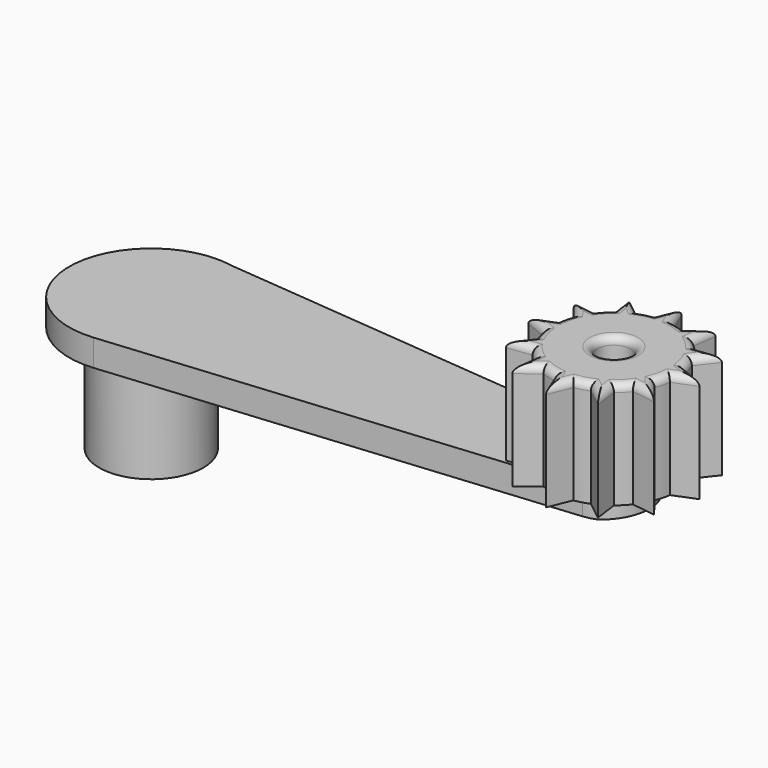
from build123d import *

# Parameters (mm, degrees)
F1_DEPTH = 6.35
F2_R     = 4
F3_DEPTH = 25.4
F5_R     = 12.3831854663
F6_DEPTH = 25.4
F7_R     = 4
F8_DEPTH = 25.4
F9_R     = 1.778


# Not quite as in the source:
# - a fillet or chamfer that OpenCascade refuses, or shapes differently, is made with other operations: its cross-section is extruded or revolved along the edge and cut away or added


with BuildPart() as f1:
    # F0 (on Top) → F1 (new body)
    with BuildSketch(Plane.XY):
        with BuildLine():
            Line((0, 19.5379621843), (3.5827930435, 19.2066540637))
            ThreePointArc((3.5827930435, 19.2066540637), (1.7990394008, 19.4549588422), (0, 19.5379621843))
        make_face()
        with BuildLine():
            Line((110.0876327298, 9.3579360824), (3.5827930435, 19.2066540637))
            Line((3.5827930435, 19.2066540637), (0, 19.5379621843))
            ThreePointArc((0, 19.5379621843), (-19.5168552551, -0.9079247047), (1.813887741, -19.453580071))
            Line((1.8138877409, -19.453580071), (110.0876327298, -9.3579360824))
            ThreePointArc((110.0876327298, -9.3579360824), (118.6201465698, 0), (110.0876327298, 9.3579360824))
        make_face()
    extrude(amount=F1_DEPTH)

    # F2 (on face) → F3 (cut)
    with BuildSketch(Plane.XY.offset(6.35)):
        with Locations((110.0876327298, 0)):
            Circle(F2_R)
    extrude(amount=-F3_DEPTH, mode=Mode.SUBTRACT)

    # F4: chamfer of 5.08 on 1 edges, made by hand

    # F4_s1 → F4_t2 (revolve, cut)
    with BuildSketch(Plane.XZ):
        Polygon((119.1676327298, 0), (114.0876327298, 5.08), (114.0876327298, 0), align=None)
    revolve(axis=Axis((110.0876327298, 0, 0), (0, 0, 1)), mode=Mode.SUBTRACT)

    # F5 (on face) → F6 (join)
    with BuildSketch(Plane(origin=(0, 0, 0), x_dir=(1, 0, 0), z_dir=(0, 0, -1))):
        Circle(F5_R)
    extrude(amount=F6_DEPTH)


with BuildPart() as f8:
    # F7 (on face) → F8 (new body)
    with BuildSketch(Plane.XY.offset(6.35)):
        with BuildLine():
            ThreePointArc((125.0559656513, -2.0569956955), (125.1614333891, -1.0309002972), (125.1966440058, 0))
            ThreePointArc((125.1966440058, 0), (125.1529244508, 1.1485674127), (125.0220188001, 2.2904878178))
            ThreePointArc((125.0220188001, 2.2904878178), (124.6508382593, 4.0243342858), (124.0790871399, 5.7027559329))
            ThreePointArc((124.0790871399, 5.7027559329), (123.1130347073, 7.656443369), (121.8759465477, 9.4508136724))
            ThreePointArc((121.8759465477, 9.4508136724), (120.687571536, 10.7667784895), (119.3532097183, 11.9344587145))
            ThreePointArc((119.3532097183, 11.9344587145), (117.5397400523, 13.143375449), (115.5712051277, 14.0788016356))
            ThreePointArc((115.5712051277, 14.0788016356), (113.8840597698, 14.624273092), (112.1446284253, 14.9683329214))
            ThreePointArc((112.1446284253, 14.9683329214), (109.9696592584, 15.1085506915), (107.797144912, 14.9343860702))
            ThreePointArc((107.797144912, 14.9343860702), (106.0632984441, 14.5632055295), (104.3848767969, 13.99145441))
            ThreePointArc((104.3848767969, 13.99145441), (102.4311893608, 13.0254019775), (100.6368190574, 11.7883138179))
            ThreePointArc((100.6368190574, 11.7883138179), (99.3208542403, 10.5999388062), (98.1531740153, 9.2655769885))
            ThreePointArc((98.1531740153, 9.2655769885), (96.9442572809, 7.4521073225), (96.0088310942, 5.4835723979))
            ThreePointArc((96.0088310942, 5.4835723979), (95.4633596378, 3.79642704), (95.1192998084, 2.0569956955))
            ThreePointArc((95.1192998084, 2.0569956955), (94.9790820383, -0.1179734715), (95.1532466596, -2.2904878178))
            ThreePointArc((95.1532466596, -2.2904878178), (95.5244272003, -4.0243342858), (96.0961783198, -5.7027559329))
            ThreePointArc((96.0961783198, -5.7027559329), (97.0622307523, -7.656443369), (98.299318912, -9.4508136724))
            ThreePointArc((98.299318912, -9.4508136724), (99.4876939236, -10.7667784895), (100.8220557413, -11.9344587145))
            ThreePointArc((100.8220557413, -11.9344587145), (102.6355254073, -13.143375449), (104.604060332, -14.0788016356))
            ThreePointArc((104.604060332, -14.0788016356), (106.2912056898, -14.624273092), (108.0306370343, -14.9683329214))
            ThreePointArc((108.0306370343, -14.9683329214), (110.2056062013, -15.1085506915), (112.3781205476, -14.9343860702))
            ThreePointArc((112.3781205476, -14.9343860702), (114.1119670156, -14.5632055295), (115.7903886627, -13.99145441))
            ThreePointArc((115.7903886627, -13.99145441), (117.7440760988, -13.0254019775), (119.5384464022, -11.7883138179))
            ThreePointArc((119.5384464022, -11.7883138179), (120.8544112194, -10.5999388062), (122.0220914443, -9.2655769885))
            ThreePointArc((122.0220914443, -9.2655769885), (123.2310081788, -7.4521073225), (124.1664343655, -5.4835723979))
            ThreePointArc((124.1664343655, -5.4835723979), (124.7119058218, -3.79642704), (125.0559656513, -2.0569956955))
        make_face()
        with Locations((110.0876327298, 0)):
            Circle(F7_R, mode=Mode.SUBTRACT)
        with BuildLine():
            ThreePointArc((125.0220188001, 2.2904878178), (125.1529244508, 1.1485674127), (125.1966440058, 0))
            ThreePointArc((125.1966440058, 0), (125.1614333891, -1.0309002972), (125.0559656513, -2.0569956955))
            Line((125.0559656513, -2.0569956955), (130.3779385678, 0.0894885204))
            Line((130.3779385678, 0.0894885204), (125.0220188001, 2.2904878178))
        make_face()
        with BuildLine():
            ThreePointArc((121.8759465477, 9.4508136724), (123.1130347073, 7.656443369), (124.0790871399, 5.7027559329))
            Line((124.0790871399, 5.7027559329), (127.6148087759, 10.222652251))
            Line((127.6148087759, 10.222652251), (121.8759465477, 9.4508136724))
        make_face()
        with BuildLine():
            Line((127.7042972963, -10.067653587), (124.1664343655, -5.4835723979))
            ThreePointArc((124.1664343655, -5.4835723979), (123.2310081788, -7.4521073225), (122.0220914443, -9.2655769885))
            Line((122.0220914443, -9.2655769885), (127.7042972963, -10.067653587))
        make_face()
        with BuildLine():
            ThreePointArc((115.5712051277, 14.0788016356), (117.5397400523, 13.143375449), (119.3532097183, 11.9344587145))
            Line((119.3532097183, 11.9344587145), (120.1552863168, 17.6166645665))
            Line((120.1552863168, 17.6166645665), (115.5712051277, 14.0788016356))
        make_face()
        with BuildLine():
            Line((120.3102849809, -17.527176046), (119.5384464022, -11.7883138179))
            ThreePointArc((119.5384464022, -11.7883138179), (117.7440760988, -13.0254019775), (115.7903886627, -13.99145441))
            Line((115.7903886627, -13.99145441), (120.3102849809, -17.527176046))
        make_face()
        with BuildLine():
            ThreePointArc((107.797144912, 14.9343860702), (109.9696592584, 15.1085506915), (112.1446284253, 14.9683329214))
            Line((112.1446284253, 14.9683329214), (109.9981442094, 20.290305838))
            Line((109.9981442094, 20.290305838), (107.797144912, 14.9343860702))
        make_face()
        with BuildLine():
            Line((110.1771212503, -20.290305838), (112.3781205476, -14.9343860702))
            ThreePointArc((112.3781205476, -14.9343860702), (110.2056062013, -15.1085506915), (108.0306370343, -14.9683329214))
            Line((108.0306370343, -14.9683329214), (110.1771212503, -20.290305838))
        make_face()
        with BuildLine():
            ThreePointArc((100.6368190574, 11.7883138179), (102.4311893608, 13.0254019775), (104.3848767969, 13.99145441))
            Line((104.3848767969, 13.99145441), (99.8649804788, 17.527176046))
            Line((99.8649804788, 17.527176046), (100.6368190574, 11.7883138179))
        make_face()
        with BuildLine():
            Line((100.0199791429, -17.6166645665), (104.604060332, -14.0788016356))
            ThreePointArc((104.604060332, -14.0788016356), (102.6355254073, -13.143375449), (100.8220557413, -11.9344587145))
            Line((100.8220557413, -11.9344587145), (100.0199791429, -17.6166645665))
        make_face()
        with BuildLine():
            ThreePointArc((96.0088310942, 5.4835723979), (96.9442572809, 7.4521073225), (98.1531740153, 9.2655769885))
            Line((98.1531740153, 9.2655769885), (92.4709681633, 10.067653587))
            Line((92.4709681633, 10.067653587), (96.0088310942, 5.4835723979))
        make_face()
        with BuildLine():
            Line((92.5604566838, -10.222652251), (98.299318912, -9.4508136724))
            ThreePointArc((98.299318912, -9.4508136724), (97.0622307523, -7.656443369), (96.0961783198, -5.7027559329))
            Line((96.0961783198, -5.7027559329), (92.5604566838, -10.222652251))
        make_face()
        with BuildLine():
            ThreePointArc((95.1532466596, -2.2904878178), (94.9790820383, -0.1179734715), (95.1192998084, 2.0569956955))
            Line((95.1192998084, 2.0569956955), (89.7973268918, -0.0894885204))
            Line((89.7973268918, -0.0894885204), (95.1532466596, -2.2904878178))
        make_face()
    extrude(amount=F8_DEPTH)

    # F9
    f9_edges = [f8.edges().sort_by_distance(p)[0] for p in [
        (127.716952, -0.983754, 31.75),
        (127.699979, 1.189988, 31.75),
        (124.650838, 4.024334, 31.75),
        (125.846948, 7.962704, 31.75),
        (124.745378, 9.836733, 31.75),
        (120.687572, 10.766778, 31.75),
        (119.754248, 14.775562, 31.75),
        (117.863246, 15.847733, 31.75),
        (113.88406, 14.624273, 31.75),
        (111.071386, 17.629319, 31.75),
        (108.897645, 17.612346, 31.75),
        (106.063298, 14.563206, 31.75),
        (102.124929, 15.759315, 31.75),
        (100.2509, 14.657745, 31.75),
        (99.320854, 10.599939, 31.75),
        (95.312071, 9.666615, 31.75),
        (94.2399, 7.775613, 31.75),
        (95.46336, 3.796427, 31.75),
        (92.458313, 0.983754, 31.75),
        (92.475287, -1.189988, 31.75),
        (95.524427, -4.024334, 31.75),
        (94.328318, -7.962704, 31.75),
        (95.429888, -9.836733, 31.75),
        (99.487694, -10.766778, 31.75),
        (100.421017, -14.775562, 31.75),
        (102.31202, -15.847733, 31.75),
        (106.291206, -14.624273, 31.75),
        (109.103879, -17.629319, 31.75),
        (111.277621, -17.612346, 31.75),
        (114.111967, -14.563206, 31.75),
        (118.050337, -15.759315, 31.75),
        (119.924366, -14.657745, 31.75),
        (120.854411, -10.599939, 31.75),
        (124.863194, -9.666615, 31.75),
        (125.935366, -7.775613, 31.75),
        (124.711906, -3.796427, 31.75),
        (106.087633, 0, 31.75),
    ]]
    fillet(f9_edges, radius=F9_R)


solid = Compound([f1.part, f8.part])
